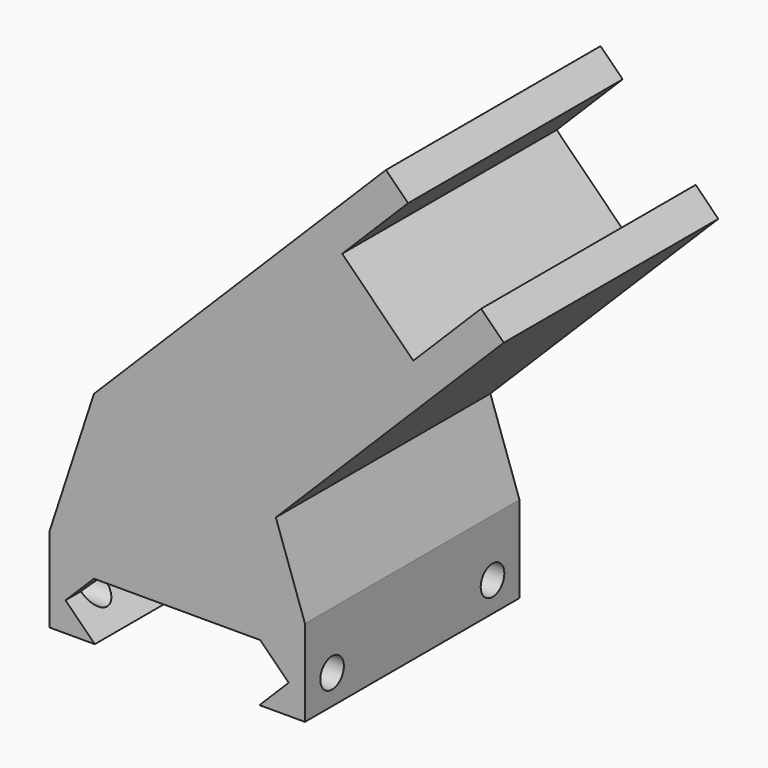
from build123d import *

# Parameters (mm, degrees)
F1_DEPTH = 25.4
F3_D     = 2.794
F3_DEPTH = 25.4
F3_TIP   = 0.8394022848
F4_D     = 2.794
F4_DEPTH = 25.4
F4_START = 10.1278152
F4_TIP   = 0.8394022848


# Not quite as in the source:
# - ends of sketch curves that miss each other by under 0.0002 mm in the source are joined


with BuildPart() as f1:
    # F0 (on Front) → F1 (new body)
    with BuildSketch(Plane.XZ):
        Polygon((11.0066256276, -6.5430273301), (8.240193387, -9.310965985), (12.5485987193, -9.310965985), (12.5485987193, -1.1086727812), (9.7906497979, 6.8444932552), (24.9488617122, 22.0027051695), (31.3820510637, 28.435894521), (29.2404852808, 30.5774603039), (22.8072959293, 24.1442709524), (16.0729033236, 30.8786635582), (22.3196721338, 37.1254323684), (20.2273843878, 39.2177201144), (14.0302290969, 33.0205648235), (13.9806155776, 32.9709513042), (-7.4406042695, 11.5497314571), (-7.4406041338, 11.5466563515), (-7.4413635659, 11.5474157835), (-11.6305711889, -1.2286720797), (-11.6305711889, -9.3063699081), (-7.3613829189, -9.3063699081), (-10.1278151595, -6.5384312532), (-7.4425795762, -3.8636476732), (8.3167760077, -3.8636476732), align=None)
    extrude(amount=F1_DEPTH)

    # F3 (one way)
    with BuildSketch(Plane(origin=(0, 0, 0), x_dir=(0, 1, 0), z_dir=(-1, 0, 0))):
        with Locations((-22.1899207681, 6.5197679214), (-3.1917574815, 6.5197679214)):
            Circle(F3_D / 2)
    extrude(amount=-F3_DEPTH, mode=Mode.SUBTRACT)
    with Locations(Plane(origin=(0, 0, 0), x_dir=(0, 1, 0), z_dir=(-1, 0, 0))):
        with Locations((-22.1899207681, 6.5197679214), (-3.1917574815, 6.5197679214)):
            with Locations((0, 0, -(F3_DEPTH + F3_TIP / 2))):  # 118° drill point
                Cone(0, F3_D / 2, F3_TIP, mode=Mode.SUBTRACT)

    # F4
    # its depths count from where the whole tool has entered the part; down to there all is cleared
    with Locations(Plane.YZ.offset(-F4_START)):
        with Locations((-3.1917574815, -6.5197679214), (-22.1899207681, -6.5197679214)):
            Hole(F4_D / 2, depth=F4_DEPTH)
            with Locations((0, 0, -(F4_DEPTH + F4_TIP / 2))):  # 118° drill point
                Cone(0, F4_D / 2, F4_TIP, mode=Mode.SUBTRACT)


with BuildPart() as f5_1:
    # F5: copy of F1
    add(f1.part)


solid = Compound([f1.part, f5_1.part])
